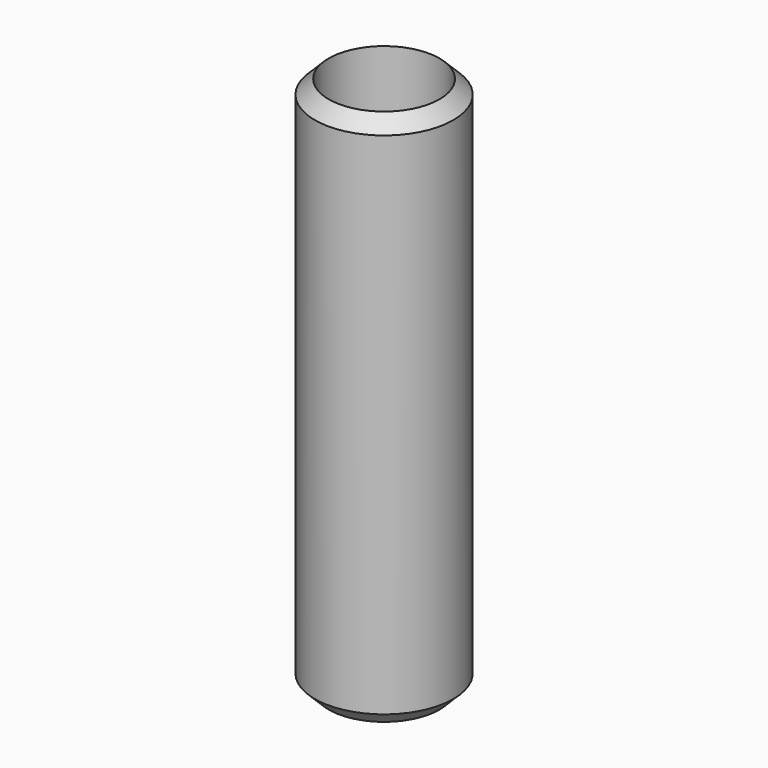
from build123d import *

# Parameters (mm, degrees)
F0_R     = 15.875
F0_R_2   = 12.7
F1_DEPTH = 127


# Not quite as in the source:
# - a fillet or chamfer that OpenCascade refuses, or shapes differently, is made with other operations: its cross-section is extruded or revolved along the edge and cut away or added


with BuildPart() as f1:
    # F0 (on Top) → F1 (new body)
    with BuildSketch(Plane.XY):
        Circle(F0_R)
        Circle(F0_R_2, mode=Mode.SUBTRACT)
    extrude(amount=F1_DEPTH)

    # F2: chamfer of 5.08 on 3 edges, made by hand

    # F2_s1 → F2_t2 (revolve, cut)
    with BuildSketch(Plane.XZ):
        Polygon((15.875, 5.08), (10.795, 0), (15.875, 0), align=None)
    revolve(axis=Axis((0, 0, 0), (0, 0, 1)), mode=Mode.SUBTRACT)

    # F2_s3 → F2_t4 (revolve, cut)
    with BuildSketch(Plane.XZ):
        Polygon((15.875, 121.92), (10.795, 127), (15.875, 127), align=None)
    revolve(axis=Axis((0, 0, 127), (0, 0, 1)), mode=Mode.SUBTRACT)


solid = f1.part
